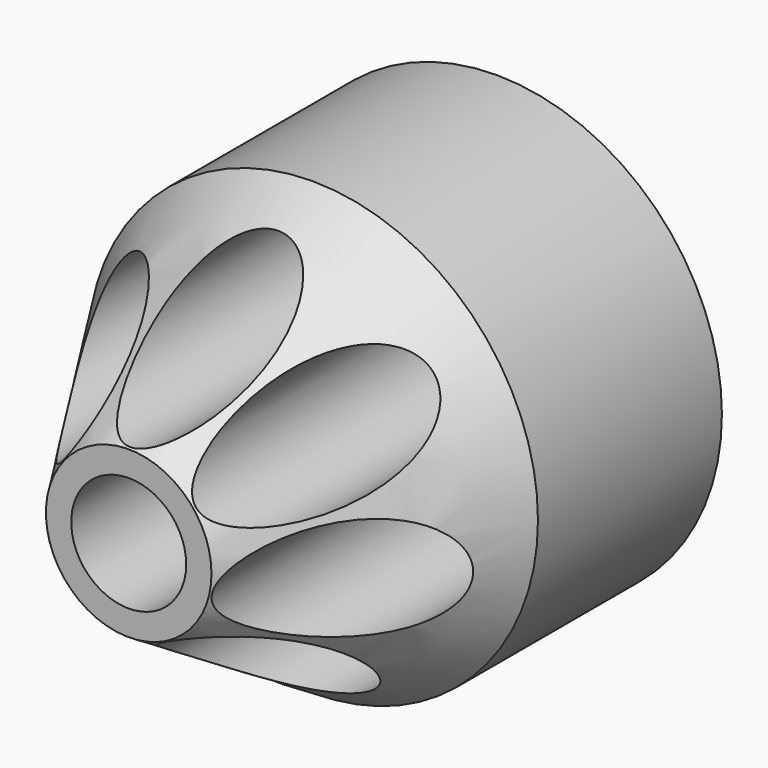
from build123d import *

# Parameters (mm, degrees)
F0_R     = 12.446
F0_R_2   = 3.175
F1_DEPTH = 25.4
F3_D     = 6.35


# Not quite as in the source:
# - a fillet or chamfer that OpenCascade refuses, or shapes differently, is made with other operations: its cross-section is extruded or revolved along the edge and cut away or added


with BuildPart() as f1:
    # F0 (on Front) → F1 (new body)
    with BuildSketch(Plane.XZ):
        Circle(F0_R)
        Circle(F0_R_2, mode=Mode.SUBTRACT)
    extrude(amount=F1_DEPTH)

    # F3 (through all)
    with Locations(Plane(origin=(0, 0, 0), x_dir=(-1, 0, 0), z_dir=(0, 1, 0))):
        with Locations((0, 7.8105), (6.1064947938, 4.8697670974), (7.6146744581, -1.7379997547), (3.3888489444, -7.0370173428), (-3.3888489444, -7.0370173428), (-7.6146744581, -1.7379997547), (-6.1064947938, 4.8697670974)):
            Hole(F3_D / 2)

    # F6: chamfer of 7.874 x 12.7 on 1 edges, made by hand

    # F6_s1 → F6_t2 (revolve, cut)
    with BuildSketch(Plane.XY):
        Polygon((12.446, -12.7), (4.572, -25.4), (12.446, -25.4), align=None)
    revolve(axis=Axis((0, -25.4, 0), (0, -1, 0)), mode=Mode.SUBTRACT)


solid = f1.part
